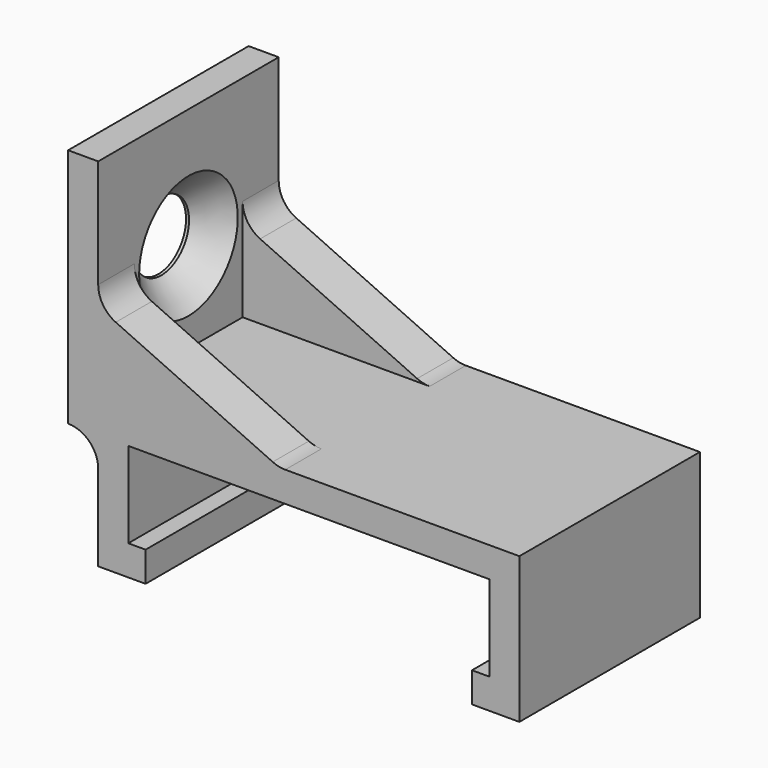
from build123d import *

# Parameters (mm, degrees)
F1_DEPTH = 7.5
F2_DEPTH = 4.5
F3_R     = 2.3
F4_DEPTH = 5
F5_SIZE  = 1.8
F6_R     = 1.99999


# Not quite as in the source:
# - a fillet or chamfer is up to 0.001 mm smaller than in the source, because OpenCascade refuses the exact size


with BuildPart() as f1:
    # F0 (on Front) → F1 (new body, symmetric)
    with BuildSketch(Plane.XZ):
        Polygon((2, 16), (0, 16), (0, 0), (2, 0), (2, -7.7), (5.15, -7.7), (5.15, -5.7), (4, -5.7), (4, 0), (28, 0), (28, -5.7), (26.85, -5.7), (26.85, -7.7), (30, -7.7), (30, 2), (14, 2), (2, 2), (2, 7.5), align=None)
        Polygon((14, 2), (2, 7.5), (2, 2), align=None)
    extrude(amount=F1_DEPTH, both=True)

    # F0 (on Front) → F2 (cut, symmetric)
    with BuildSketch(Plane.XZ):
        Polygon((14, 2), (2, 7.5), (2, 2), align=None)
    extrude(amount=F2_DEPTH, both=True, mode=Mode.SUBTRACT)

    # F3 (on face) → F4 (cut)
    with BuildSketch(Plane(origin=(0, 0, 0), x_dir=(0, -1, 0), z_dir=(-1, 0, 0))):
        with Locations((0, 8)):
            Circle(F3_R)
    extrude(amount=-F4_DEPTH, mode=Mode.SUBTRACT)

    # F5
    f5_edges = [f1.edges().sort_by_distance(p)[0] for p in [
        (2, 2.3, 8),
    ]]
    chamfer(f5_edges, length=F5_SIZE)

    # F6 (radius 2 in the source; OpenCascade refuses exactly that, so slightly less here)
    f6_edges = [f1.edges().sort_by_distance(p)[0] for p in [
        (2, -6, 7.5),
        (14, 6, 2),
        (14, -6, 2),
        (2, 6, 7.5),
        (2, 0, 0),
    ]]
    fillet(f6_edges, radius=F6_R)


solid = f1.part
